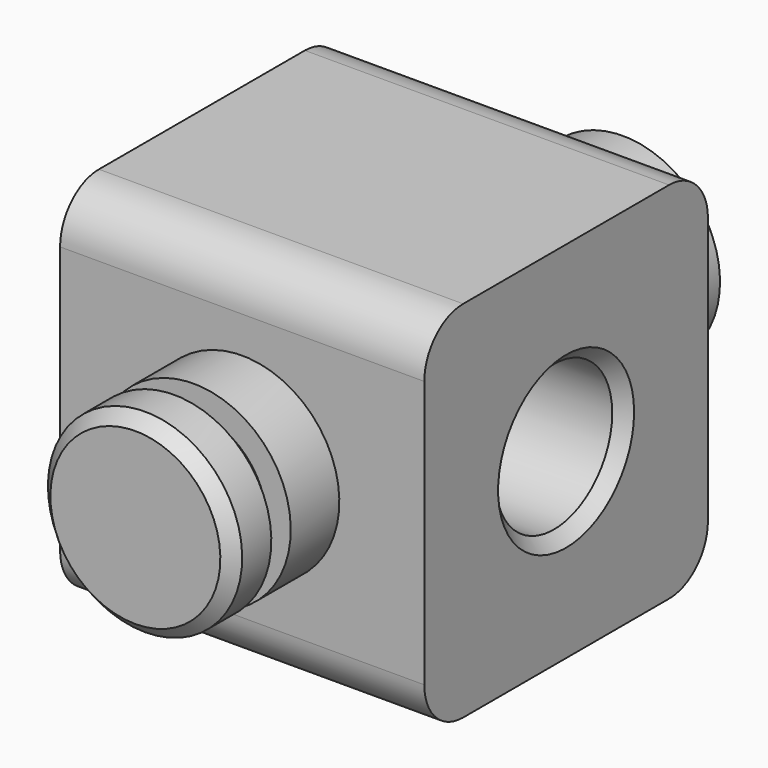
from build123d import *

# Parameters (mm, degrees)
F0_W     = 14.6
F0_H     = 15
F1_DEPTH = 15
F2_R     = 2
F3_R     = 3
F4_DEPTH = 15.001
F5_SIZE2 = 0.5
F5_SIZE  = 0.5
F9_SIZE2 = 0.5
F9_SIZE  = 0.5


# Not quite as in the source:
# - a pattern or mirror of a feature is missing from the dataset's text; its kind, count and spacing are read off the source's solid


with BuildPart() as f1:
    # F0 (on Right) → F1 (new body)
    with BuildSketch(Plane.YZ):
        Rectangle(F0_W, F0_H)
    extrude(amount=-F1_DEPTH)

    # F2
    f2_edges = [f1.edges().sort_by_distance(p)[0] for p in [
        (-7.5, -7.3, 7.5),
        (-7.5, 7.3, 7.5),
        (-7.5, -7.3, -7.5),
        (-7.5, 7.3, -7.5),
    ]]
    fillet(f2_edges, radius=F2_R)

    # F3 (on face) → F4 (cut, through all)
    with BuildSketch(Plane.YZ):
        Circle(F3_R)
    extrude(amount=-F4_DEPTH, mode=Mode.SUBTRACT)

    # F5
    f5_edges = [f1.edges().sort_by_distance(p)[0] for p in [
        (0, -3, 0),
        (-7.5, 3, 0),
        (-15, -3, 0),
    ]]
    chamfer(f5_edges, length=F5_SIZE, length2=F5_SIZE2)

    # F7 (on mid) → F8 (revolve)
    with BuildSketch(Plane.YZ.offset(-7.5)):
        Polygon((-7.3, 0), (-12.8, 0), (-12.8, -4), (-10.8, -4), (-10.8, -3), (-9.8, -3), (-9.8, -4), (-7.3, -4), align=None)
    f8 = revolve(axis=Axis((-7.5, -3.65, 0), (0, -1, 0)))

    # F8_copies: F8 across plane
    add(f8.mirror(Plane.ZX))

    # F9
    f9_edges = [f1.edges().sort_by_distance(p)[0] for p in [
        (-7.5, -12.8, 4),
        (-7.5, 12.8, 4),
    ]]
    chamfer(f9_edges, length=F9_SIZE, length2=F9_SIZE2)


solid = f1.part
